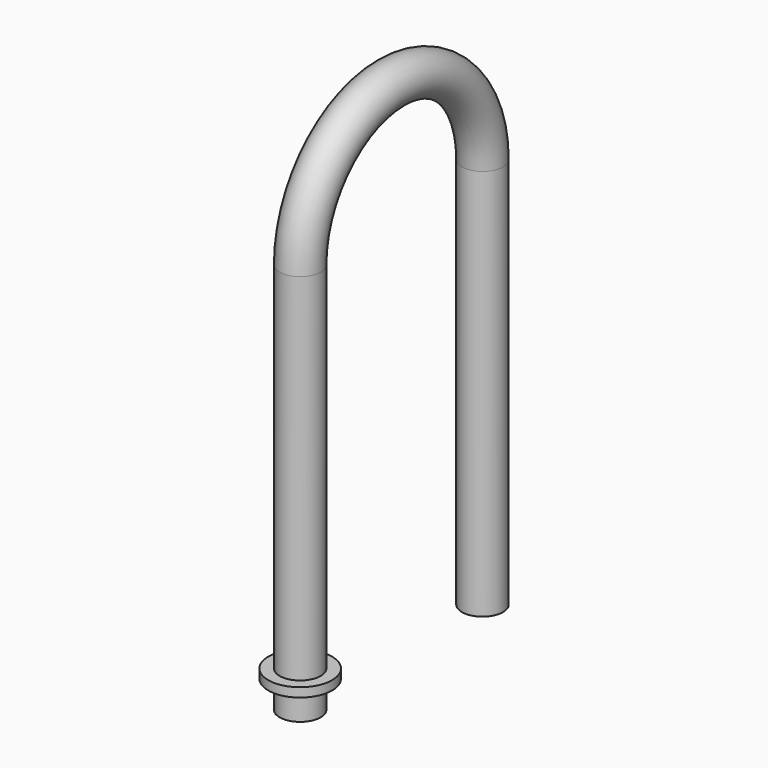
from build123d import *

# Parameters (mm, degrees)
F1_R     = 5.715
F1_R_2   = 3.81
F4_R     = 8.89
F4_R_2   = 4.360362463
F5_DEPTH = 2.54


with BuildPart() as f2:
    # F2: sweep along a path in F0
    with BuildLine(Plane.YZ) as f2_path:
        Line((31.75, -109.22), (31.75, 0))
        ThreePointArc((31.75, 0), (0, 31.75), (-31.75, 0))
        Line((-31.75, 0), (-31.75, -109.22))
    # F1 (on Top) → F2 (sweep)
    with BuildSketch(Plane.XY):
        with Locations((0, -31.75)):
            Circle(F1_R)
        with Locations((0, -31.75)):
            Circle(F1_R_2, mode=Mode.SUBTRACT)
    sweep(path=f2_path.line)

    # F4 (on offset) → F5 (join)
    with BuildSketch(Plane.XY.offset(-101.6)):
        with Locations((0, -31.75)):
            Circle(F4_R)
        with Locations((0, -31.75)):
            Circle(F4_R_2, mode=Mode.SUBTRACT)
    extrude(amount=F5_DEPTH)


solid = f2.part
